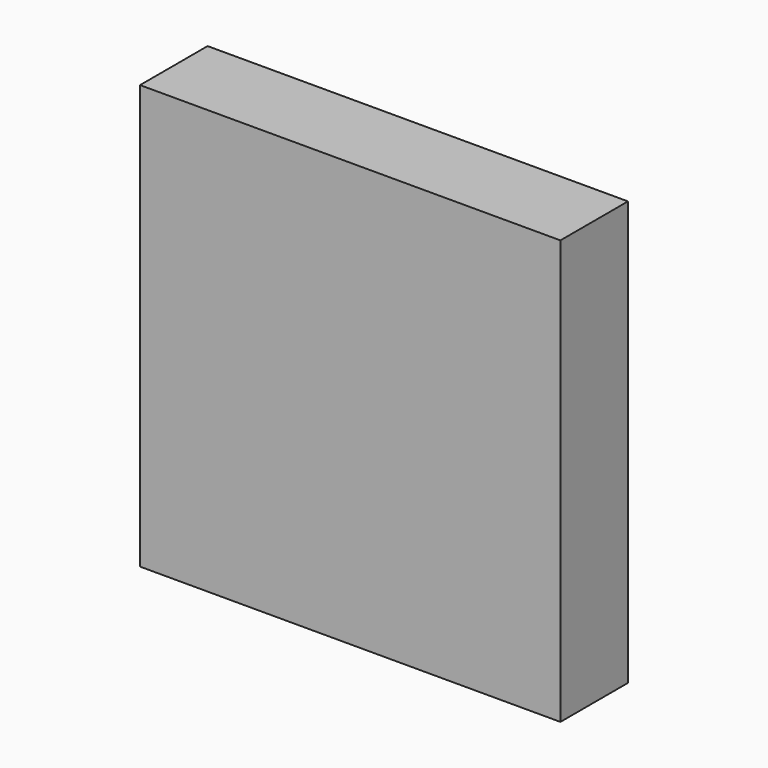
from build123d import *

# Parameters (mm, degrees)
F0_W     = 149.2990702391
F0_H     = 150.5607590079
F1_DEPTH = 30


# Not quite as in the source:
# - the program builds the solid bodies; features that only make, move or delete a surface that nothing else refers to are left out


with BuildPart() as f1:
    # F0 (on Front) → F1 (new body)
    with BuildSketch(Plane.XZ):
        with Locations((-0.1051425934, -0.2102814615)):
            Rectangle(F0_W, F0_H)
    extrude(amount=-F1_DEPTH)


solid = f1.part
